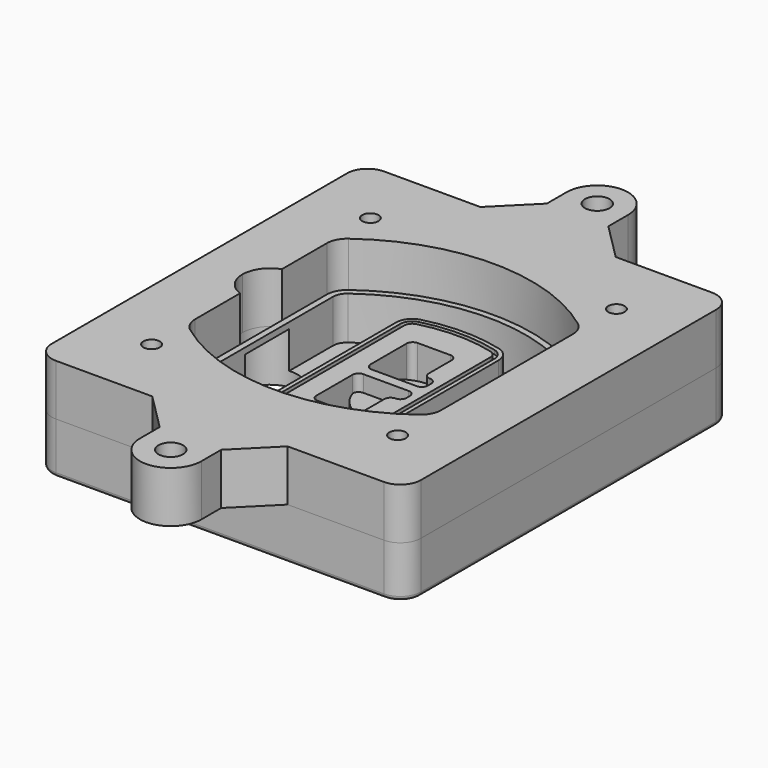
from build123d import *

# Parameters (mm, degrees)
F0_R      = 4
F1_DEPTH  = 25
F2_DEPTH  = 3
F3_DEPTH  = 18
F5_DEPTH  = 21
F6_DEPTH  = 2
F8_DEPTH  = 20
F9_DEPTH  = 16
F10_DEPTH = 25
F7_R      = 6
F7_R_2    = 4
F11_DEPTH = 6
F13_DEPTH = 9
F15_R     = 2
F16_R     = 4
F16_R_2   = 6
F17_DEPTH = 25


# Not quite as in the source:
# - a feature of the source that left no trace in its solid (it failed there, or was rolled back) is left out
# - a feature names something its author has since deleted; it is built from what else it names


with BuildPart() as f1:
    # F0 (on Top) → F1 (new body)
    with BuildSketch(Plane.XY):
        with BuildLine():
            ThreePointArc((-90, -90), (-87.0710678119, -97.0710678119), (-80, -100))
            Line((-80, -100), (80, -100))
            ThreePointArc((80, -100), (87.0710678119, -97.0710678119), (90, -90))
            Line((90, -90), (90, 90))
            ThreePointArc((90, 90), (87.0710678119, 97.0710678119), (80, 100))
            Line((80, 100), (-80, 100))
            ThreePointArc((-80, 100), (-87.0710678119, 97.0710678119), (-90, 90))
            Line((-90, 90), (-90, -90))
        make_face()
        with Locations((-60, -66.6666666667)):
            Circle(F0_R, mode=Mode.SUBTRACT)
        with Locations((60, -66.6666666667)):
            Circle(F0_R, mode=Mode.SUBTRACT)
        with Locations((-60, 66.6666666667)):
            Circle(F0_R, mode=Mode.SUBTRACT)
        with BuildLine():
            ThreePointArc((-64, 40.142841612), (-62.5058275186, 46.4360346072), (-58.3422459893, 51.3859253461))
            ThreePointArc((-58.3422459893, 51.3859253461), (0, 70.6666666667), (58.3422459893, 51.3859253461))
            ThreePointArc((58.3422459893, 51.3859253461), (62.5058275186, 46.4360346072), (64, 40.142841612))
            Line((64, 40.142841612), (64, -40.142841612))
            ThreePointArc((64, -40.142841612), (62.5058275186, -46.4360346072), (58.3422459893, -51.3859253461))
            ThreePointArc((58.3422459893, -51.3859253461), (0, -70.6666666667), (-58.3422459893, -51.3859253461))
            ThreePointArc((-58.3422459893, -51.3859253461), (-62.5058275186, -46.4360346072), (-64, -40.142841612))
            Line((-64, -40.142841612), (-64, 40.142841612))
        make_face(mode=Mode.SUBTRACT)
        with Locations((60, 66.6666666667)):
            Circle(F0_R, mode=Mode.SUBTRACT)
        with BuildLine():
            ThreePointArc((58.3422459893, 51.3859253461), (0, 70.6666666667), (-58.3422459893, 51.3859253461))
            ThreePointArc((-58.3422459893, 51.3859253461), (-62.5058275186, 46.4360346072), (-64, 40.142841612))
            Line((-64, 40.142841612), (-64, -40.142841612))
            ThreePointArc((-64, -40.142841612), (-62.5058275186, -46.4360346072), (-58.3422459893, -51.3859253461))
            ThreePointArc((-58.3422459893, -51.3859253461), (0, -70.6666666667), (58.3422459893, -51.3859253461))
            ThreePointArc((58.3422459893, -51.3859253461), (62.5058275186, -46.4360346072), (64, -40.142841612))
            Line((64, -40.142841612), (64, 40.142841612))
            ThreePointArc((64, 40.142841612), (62.5058275186, 46.4360346072), (58.3422459893, 51.3859253461))
        make_face()
        with BuildLine():
            Line((-60, -40.142841612), (-60, 40.142841612))
            ThreePointArc((-60, 40.142841612), (-58.9327339419, 44.6379794657), (-55.9587471352, 48.1736157078))
            ThreePointArc((-55.9587471352, 48.1736157078), (0, 66.6666666667), (55.9587471352, 48.1736157078))
            ThreePointArc((55.9587471352, 48.1736157078), (58.9327339419, 44.6379794657), (60, 40.142841612))
            Line((60, 40.142841612), (60, -40.142841612))
            ThreePointArc((60, -40.142841612), (58.9327339419, -44.6379794657), (55.9587471352, -48.1736157078))
            ThreePointArc((55.9587471352, -48.1736157078), (0, -66.6666666667), (-55.9587471352, -48.1736157078))
            ThreePointArc((-55.9587471352, -48.1736157078), (-58.9327339419, -44.6379794657), (-60, -40.142841612))
        make_face(mode=Mode.SUBTRACT)
        with BuildLine():
            ThreePointArc((-55.9587471352, 48.1736157078), (-58.9327339419, 44.6379794657), (-60, 40.142841612))
            Line((-60, 40.142841612), (-60, -40.142841612))
            ThreePointArc((-60, -40.142841612), (-58.9327339419, -44.6379794657), (-55.9587471352, -48.1736157078))
            ThreePointArc((-55.9587471352, -48.1736157078), (0, -66.6666666667), (55.9587471352, -48.1736157078))
            ThreePointArc((55.9587471352, -48.1736157078), (58.9327339419, -44.6379794657), (60, -40.142841612))
            Line((60, -40.142841612), (60, 40.142841612))
            ThreePointArc((60, 40.142841612), (58.9327339419, 44.6379794657), (55.9587471352, 48.1736157078))
            ThreePointArc((55.9587471352, 48.1736157078), (0, 66.6666666667), (-55.9587471352, 48.1736157078))
        make_face()
        with BuildLine():
            ThreePointArc((54.1711229947, 45.764383479), (56.2529137593, 43.2894381096), (57, 40.142841612))
            Line((57, 40.142841612), (57, -40.142841612))
            ThreePointArc((57, -40.142841612), (56.2529137593, -43.2894381096), (54.1711229947, -45.764383479))
            ThreePointArc((54.1711229947, -45.764383479), (0, -63.6666666667), (-54.1711229947, -45.764383479))
            ThreePointArc((-54.1711229947, -45.764383479), (-56.2529137593, -43.2894381096), (-57, -40.142841612))
            Line((-57, -40.142841612), (-57, 40.142841612))
            ThreePointArc((-57, 40.142841612), (-56.2529137593, 43.2894381096), (-54.1711229947, 45.764383479))
            ThreePointArc((-54.1711229947, 45.764383479), (0, 63.6666666667), (54.1711229947, 45.764383479))
        make_face(mode=Mode.SUBTRACT)
        with BuildLine():
            Line((57, -40.142841612), (57, 40.142841612))
            ThreePointArc((57, 40.142841612), (56.2529137593, 43.2894381096), (54.1711229947, 45.764383479))
            ThreePointArc((54.1711229947, 45.764383479), (0, 63.6666666667), (-54.1711229947, 45.764383479))
            ThreePointArc((-54.1711229947, 45.764383479), (-56.2529137593, 43.2894381096), (-57, 40.142841612))
            Line((-57, 40.142841612), (-57, -40.142841612))
            ThreePointArc((-57, -40.142841612), (-56.2529137593, -43.2894381096), (-54.1711229947, -45.764383479))
            ThreePointArc((-54.1711229947, -45.764383479), (0, -63.6666666667), (54.1711229947, -45.764383479))
            ThreePointArc((54.1711229947, -45.764383479), (56.2529137593, -43.2894381096), (57, -40.142841612))
        make_face()
    extrude(amount=-F1_DEPTH)

    # F0 (on Top) → F2 (join)
    with BuildSketch(Plane.XY):
        with BuildLine():
            ThreePointArc((-55.9587471352, 48.1736157078), (-58.9327339419, 44.6379794657), (-60, 40.142841612))
            Line((-60, 40.142841612), (-60, -40.142841612))
            ThreePointArc((-60, -40.142841612), (-58.9327339419, -44.6379794657), (-55.9587471352, -48.1736157078))
            ThreePointArc((-55.9587471352, -48.1736157078), (0, -66.6666666667), (55.9587471352, -48.1736157078))
            ThreePointArc((55.9587471352, -48.1736157078), (58.9327339419, -44.6379794657), (60, -40.142841612))
            Line((60, -40.142841612), (60, 40.142841612))
            ThreePointArc((60, 40.142841612), (58.9327339419, 44.6379794657), (55.9587471352, 48.1736157078))
            ThreePointArc((55.9587471352, 48.1736157078), (0, 66.6666666667), (-55.9587471352, 48.1736157078))
        make_face()
        with BuildLine():
            ThreePointArc((54.1711229947, 45.764383479), (56.2529137593, 43.2894381096), (57, 40.142841612))
            Line((57, 40.142841612), (57, -40.142841612))
            ThreePointArc((57, -40.142841612), (56.2529137593, -43.2894381096), (54.1711229947, -45.764383479))
            ThreePointArc((54.1711229947, -45.764383479), (0, -63.6666666667), (-54.1711229947, -45.764383479))
            ThreePointArc((-54.1711229947, -45.764383479), (-56.2529137593, -43.2894381096), (-57, -40.142841612))
            Line((-57, -40.142841612), (-57, 40.142841612))
            ThreePointArc((-57, 40.142841612), (-56.2529137593, 43.2894381096), (-54.1711229947, 45.764383479))
            ThreePointArc((-54.1711229947, 45.764383479), (0, 63.6666666667), (54.1711229947, 45.764383479))
        make_face(mode=Mode.SUBTRACT)
    extrude(amount=F2_DEPTH)

    # F0 (on Top) → F3 (cut)
    with BuildSketch(Plane.XY):
        with BuildLine():
            Line((57, -40.142841612), (57, 40.142841612))
            ThreePointArc((57, 40.142841612), (56.2529137593, 43.2894381096), (54.1711229947, 45.764383479))
            ThreePointArc((54.1711229947, 45.764383479), (0, 63.6666666667), (-54.1711229947, 45.764383479))
            ThreePointArc((-54.1711229947, 45.764383479), (-56.2529137593, 43.2894381096), (-57, 40.142841612))
            Line((-57, 40.142841612), (-57, -40.142841612))
            ThreePointArc((-57, -40.142841612), (-56.2529137593, -43.2894381096), (-54.1711229947, -45.764383479))
            ThreePointArc((-54.1711229947, -45.764383479), (0, -63.6666666667), (54.1711229947, -45.764383479))
            ThreePointArc((54.1711229947, -45.764383479), (56.2529137593, -43.2894381096), (57, -40.142841612))
        make_face()
    extrude(amount=-F3_DEPTH, mode=Mode.SUBTRACT)

    # F4 (on face) → F5 (join, through all)
    with BuildSketch(Plane.XY.offset(3)):
        with BuildLine():
            ThreePointArc((-25, -38.5044362778), (-23.3253910568, -43.402336642), (-19.0026430055, -46.2497200681))
            ThreePointArc((-19.0026430055, -46.2497200681), (0, -48.6666666667), (19.0026430055, -46.2497200681))
            ThreePointArc((19.0026430055, -46.2497200681), (23.3253910568, -43.402336642), (25, -38.5044362778))
            Line((25, -38.5044362778), (25, 38.5044362778))
            ThreePointArc((25, 38.5044362778), (23.3253910568, 43.402336642), (19.0026430055, 46.2497200681))
            ThreePointArc((19.0026430055, 46.2497200681), (0, 48.6666666667), (-19.0026430055, 46.2497200681))
            ThreePointArc((-19.0026430055, 46.2497200681), (-23.3253910568, 43.402336642), (-25, 38.5044362778))
            Line((-25, 38.5044362778), (-25, -38.5044362778))
        make_face()
        with BuildLine():
            ThreePointArc((18.5019822541, 44.3133991205), (21.7440432926, 42.177861551), (23, 38.5044362778))
            Line((23, 38.5044362778), (23, -38.5044362778))
            ThreePointArc((23, -38.5044362778), (21.7440432926, -42.177861551), (18.5019822541, -44.3133991205))
            ThreePointArc((18.5019822541, -44.3133991205), (0, -46.6666666667), (-18.5019822541, -44.3133991205))
            ThreePointArc((-18.5019822541, -44.3133991205), (-21.7440432926, -42.177861551), (-23, -38.5044362778))
            Line((-23, -38.5044362778), (-23, 38.5044362778))
            ThreePointArc((-23, 38.5044362778), (-21.7440432926, 42.177861551), (-18.5019822541, 44.3133991205))
            ThreePointArc((-18.5019822541, 44.3133991205), (0, 46.6666666667), (18.5019822541, 44.3133991205))
        make_face(mode=Mode.SUBTRACT)
        with BuildLine():
            Line((23, -38.5044362778), (23, 38.5044362778))
            ThreePointArc((23, 38.5044362778), (21.7440432926, 42.177861551), (18.5019822541, 44.3133991205))
            ThreePointArc((18.5019822541, 44.3133991205), (0, 46.6666666667), (-18.5019822541, 44.3133991205))
            ThreePointArc((-18.5019822541, 44.3133991205), (-21.7440432926, 42.177861551), (-23, 38.5044362778))
            Line((-23, 38.5044362778), (-23, -38.5044362778))
            ThreePointArc((-23, -38.5044362778), (-21.7440432926, -42.177861551), (-18.5019822541, -44.3133991205))
            ThreePointArc((-18.5019822541, -44.3133991205), (0, -46.6666666667), (18.5019822541, -44.3133991205))
            ThreePointArc((18.5019822541, -44.3133991205), (21.7440432926, -42.177861551), (23, -38.5044362778))
        make_face()
        with BuildLine():
            ThreePointArc((18.0013215027, 42.3770781729), (20.1626955284, 40.9533864599), (21, 38.5044362778))
            Line((21, 38.5044362778), (21, -38.5044362778))
            ThreePointArc((21, -38.5044362778), (20.1626955284, -40.9533864599), (18.0013215027, -42.3770781729))
            ThreePointArc((18.0013215027, -42.3770781729), (0, -44.6666666667), (-18.0013215027, -42.3770781729))
            ThreePointArc((-18.0013215027, -42.3770781729), (-20.1626955284, -40.9533864599), (-21, -38.5044362778))
            Line((-21, -38.5044362778), (-21, 38.5044362778))
            ThreePointArc((-21, 38.5044362778), (-20.1626955284, 40.9533864599), (-18.0013215027, 42.3770781729))
            ThreePointArc((-18.0013215027, 42.3770781729), (0, 44.6666666667), (18.0013215027, 42.3770781729))
        make_face(mode=Mode.SUBTRACT)
        with BuildLine():
            Line((21, -38.5044362778), (21, 38.5044362778))
            ThreePointArc((21, 38.5044362778), (20.1626955284, 40.9533864599), (18.0013215027, 42.3770781729))
            ThreePointArc((18.0013215027, 42.3770781729), (0, 44.6666666667), (-18.0013215027, 42.3770781729))
            ThreePointArc((-18.0013215027, 42.3770781729), (-20.1626955284, 40.9533864599), (-21, 38.5044362778))
            Line((-21, 38.5044362778), (-21, -38.5044362778))
            ThreePointArc((-21, -38.5044362778), (-20.1626955284, -40.9533864599), (-18.0013215027, -42.3770781729))
            ThreePointArc((-18.0013215027, -42.3770781729), (0, -44.6666666667), (18.0013215027, -42.3770781729))
            ThreePointArc((18.0013215027, -42.3770781729), (20.1626955284, -40.9533864599), (21, -38.5044362778))
        make_face()
        with BuildLine():
            Line((-8, -2.5), (14, -2.5))
            ThreePointArc((14, -2.5), (16.1213203436, -3.3786796564), (17, -5.5))
            Line((17, -5.5), (17, -7.5))
            ThreePointArc((17, -7.5), (16.1213203436, -9.6213203436), (14, -10.5))
            ThreePointArc((14, -10.5), (11.8786796564, -11.3786796564), (11, -13.5))
            Line((11, -13.5), (11, -27.5))
            ThreePointArc((11, -27.5), (10.1213203436, -29.6213203436), (8, -30.5))
            Line((8, -30.5), (-8, -30.5))
            ThreePointArc((-8, -30.5), (-10.1213203436, -29.6213203436), (-11, -27.5))
            Line((-11, -27.5), (-11, -5.5))
            ThreePointArc((-11, -5.5), (-10.1213203436, -3.3786796564), (-8, -2.5))
        make_face(mode=Mode.SUBTRACT)
        with BuildLine():
            ThreePointArc((-8, 2.5), (-10.1213203436, 3.3786796564), (-11, 5.5))
            Line((-11, 5.5), (-11, 27.5))
            ThreePointArc((-11, 27.5), (-10.1213203436, 29.6213203436), (-8, 30.5))
            Line((-8, 30.5), (8, 30.5))
            ThreePointArc((8, 30.5), (10.1213203436, 29.6213203436), (11, 27.5))
            Line((11, 27.5), (11, 13.5))
            ThreePointArc((11, 13.5), (11.8786796564, 11.3786796564), (14, 10.5))
            ThreePointArc((14, 10.5), (16.1213203436, 9.6213203436), (17, 7.5))
            Line((17, 7.5), (17, 5.5))
            ThreePointArc((17, 5.5), (16.1213203436, 3.3786796564), (14, 2.5))
            Line((14, 2.5), (-8, 2.5))
        make_face(mode=Mode.SUBTRACT)
    extrude(amount=-F5_DEPTH)

    # F4 (on face) → F6 (cut)
    with BuildSketch(Plane.XY.offset(3)):
        with BuildLine():
            Line((23, -38.5044362778), (23, 38.5044362778))
            ThreePointArc((23, 38.5044362778), (21.7440432926, 42.177861551), (18.5019822541, 44.3133991205))
            ThreePointArc((18.5019822541, 44.3133991205), (0, 46.6666666667), (-18.5019822541, 44.3133991205))
            ThreePointArc((-18.5019822541, 44.3133991205), (-21.7440432926, 42.177861551), (-23, 38.5044362778))
            Line((-23, 38.5044362778), (-23, -38.5044362778))
            ThreePointArc((-23, -38.5044362778), (-21.7440432926, -42.177861551), (-18.5019822541, -44.3133991205))
            ThreePointArc((-18.5019822541, -44.3133991205), (0, -46.6666666667), (18.5019822541, -44.3133991205))
            ThreePointArc((18.5019822541, -44.3133991205), (21.7440432926, -42.177861551), (23, -38.5044362778))
        make_face()
        with BuildLine():
            ThreePointArc((18.0013215027, 42.3770781729), (20.1626955284, 40.9533864599), (21, 38.5044362778))
            Line((21, 38.5044362778), (21, -38.5044362778))
            ThreePointArc((21, -38.5044362778), (20.1626955284, -40.9533864599), (18.0013215027, -42.3770781729))
            ThreePointArc((18.0013215027, -42.3770781729), (0, -44.6666666667), (-18.0013215027, -42.3770781729))
            ThreePointArc((-18.0013215027, -42.3770781729), (-20.1626955284, -40.9533864599), (-21, -38.5044362778))
            Line((-21, -38.5044362778), (-21, 38.5044362778))
            ThreePointArc((-21, 38.5044362778), (-20.1626955284, 40.9533864599), (-18.0013215027, 42.3770781729))
            ThreePointArc((-18.0013215027, 42.3770781729), (0, 44.6666666667), (18.0013215027, 42.3770781729))
        make_face(mode=Mode.SUBTRACT)
    extrude(amount=-F6_DEPTH, mode=Mode.SUBTRACT)

    # F7 (on face) → F8 (join)
    with BuildSketch(Plane(origin=(0, 0, -25), x_dir=(1, 0, 0), z_dir=(0, 0, -1))):
        with BuildLine():
            ThreePointArc((-6.71157564, 0), (6.7567035675, 13.4682792075), (20.224982775, 0))
            Line((20.224982775, 0), (25.224982775, 0))
            ThreePointArc((25.224982775, 0), (6.7567035675, 18.4682792075), (-11.71157564, 0))
            Line((-11.71157564, 0), (-6.71157564, 0))
        make_face()
        with BuildLine():
            Line((-6.71157564, 0), (20.224982775, 0))
            ThreePointArc((20.224982775, 0), (6.7567035675, 13.4682792075), (-6.71157564, 0))
        make_face()
        with BuildLine():
            ThreePointArc((-6.71157564, 0), (6.7567035675, -13.4682792075), (20.224982775, 0))
            Line((20.224982775, 0), (-6.71157564, 0))
        make_face()
        with BuildLine():
            Line((25.224982775, 0), (20.224982775, 0))
            ThreePointArc((20.224982775, 0), (6.7567035675, -13.4682792075), (-6.71157564, 0))
            Line((-6.71157564, 0), (-11.71157564, 0))
            ThreePointArc((-11.71157564, 0), (6.7567035675, -18.4682792075), (25.224982775, 0))
        make_face()
    extrude(amount=-F8_DEPTH)

    # F7 (on face) → F9 (cut)
    with BuildSketch(Plane(origin=(0, 0, -25), x_dir=(1, 0, 0), z_dir=(0, 0, -1))):
        with BuildLine():
            Line((-6.71157564, 0), (20.224982775, 0))
            ThreePointArc((20.224982775, 0), (6.7567035675, 13.4682792075), (-6.71157564, 0))
        make_face()
        with BuildLine():
            ThreePointArc((-6.71157564, 0), (6.7567035675, -13.4682792075), (20.224982775, 0))
            Line((20.224982775, 0), (-6.71157564, 0))
        make_face()
    extrude(amount=-F9_DEPTH, mode=Mode.SUBTRACT)

    # F7 (on face) → F10 (cut)
    with BuildSketch(Plane(origin=(0, 0, -25), x_dir=(1, 0, 0), z_dir=(0, 0, -1))):
        with BuildLine():
            Line((-69.0318229325, 0), (-42.0952645175, 0))
            ThreePointArc((-42.0952645175, 0), (-55.563543725, 13.4682792075), (-69.0318229325, 0))
        make_face()
        with BuildLine():
            ThreePointArc((-69.0318229325, 0), (-55.563543725, -13.4682792075), (-42.0952645175, 0))
            Line((-42.0952645175, 0), (-69.0318229325, 0))
        make_face()
    extrude(amount=-F10_DEPTH, mode=Mode.SUBTRACT)

    # F7 (on face) → F11 (cut)
    with BuildSketch(Plane(origin=(0, 0, -25), x_dir=(1, 0, 0), z_dir=(0, 0, -1))):
        with Locations((60, -66.6666666667)):
            Circle(F7_R)
        with Locations((60, -66.6666666667)):
            Circle(F7_R_2, mode=Mode.SUBTRACT)
        with Locations((-60, -66.6666666667)):
            Circle(F7_R)
        with Locations((-60, -66.6666666667)):
            Circle(F7_R_2, mode=Mode.SUBTRACT)
        with Locations((-60, 66.6666666667)):
            Circle(F7_R)
        with Locations((-60, 66.6666666667)):
            Circle(F7_R_2, mode=Mode.SUBTRACT)
        with Locations((60, 66.6666666667)):
            Circle(F7_R)
        with Locations((60, 66.6666666667)):
            Circle(F7_R_2, mode=Mode.SUBTRACT)
    extrude(amount=-F11_DEPTH, mode=Mode.SUBTRACT)

    # F12 (on face) → F13 (cut, through all)
    with BuildSketch(Plane(origin=(0, 0, -9), x_dir=(1, 0, 0), z_dir=(0, 0, -1))):
        with BuildLine():
            ThreePointArc((20.224982775, 0), (20.1663399806, 1.2554664788), (19.9909222755, 2.5))
            Line((19.9909222755, 2.5), (14, 2.5))
            ThreePointArc((14, 2.5), (16.1213203436, 3.3786796564), (17, 5.5))
            Line((17, 5.5), (17, 7.5))
            ThreePointArc((17, 7.5), (16.1213203436, 9.6213203436), (14, 10.5))
            ThreePointArc((14, 10.5), (12.1627255951, 11.1284134507), (11.0951631559, 12.750384826))
            ThreePointArc((11.0951631559, 12.750384826), (11.0476113807, 12.7664660322), (11, 12.7823698976))
            Line((11, 12.7823698976), (11, -12.7823698976))
            ThreePointArc((11, -12.7823698976), (11.0476113807, -12.7664660322), (11.0951631559, -12.750384826))
            ThreePointArc((11.0951631559, -12.750384826), (12.1627255951, -11.1284134507), (14, -10.5))
            ThreePointArc((14, -10.5), (16.1213203436, -9.6213203436), (17, -7.5))
            Line((17, -7.5), (17, -5.5))
            ThreePointArc((17, -5.5), (16.1213203436, -3.3786796564), (14, -2.5))
            Line((14, -2.5), (19.9909222755, -2.5))
            ThreePointArc((19.9909222755, -2.5), (20.1663399806, -1.2554664788), (20.224982775, 0))
        make_face()
    extrude(amount=F13_DEPTH, mode=Mode.SUBTRACT)

    # F15
    f15_edges = [f1.edges().sort_by_distance(p)[0] for p in [
        (0, -100, -25),
        (-87.071068, -97.071068, -25),
        (-90, 0, -25),
        (-87.071068, 97.071068, -25),
        (87.071068, -97.071068, -25),
        (0, 100, -25),
        (90, 0, -25),
        (87.071068, 97.071068, -25),
    ]]
    fillet(f15_edges, radius=F15_R)


with BuildPart() as f17:
    # F16 (on face) → F17 (new body)
    with BuildSketch(Plane.XY):
        with BuildLine():
            Line((33, 100), (-33, 100))
            Line((-33, 100), (-80, 100))
            ThreePointArc((-80, 100), (-87.0710678119, 97.0710678119), (-90, 90))
            Line((-90, 90), (-90, -90))
            ThreePointArc((-90, -90), (-87.0710678119, -97.0710678119), (-80, -100))
            Line((-80, -100), (-33, -100))
            Line((-33, -100), (33, -100))
            Line((33, -100), (80, -100))
            ThreePointArc((80, -100), (87.0710678119, -97.0710678119), (90, -90))
            Line((90, -90), (90, 90))
            ThreePointArc((90, 90), (87.0710678119, 97.0710678119), (80, 100))
            Line((80, 100), (33, 100))
        make_face()
        with Locations((-60, -66.6666666667)):
            Circle(F16_R, mode=Mode.SUBTRACT)
        with Locations((60, -66.6666666667)):
            Circle(F16_R, mode=Mode.SUBTRACT)
        with Locations((-60, 66.6666666667)):
            Circle(F16_R, mode=Mode.SUBTRACT)
        with BuildLine():
            ThreePointArc((-60, 40.142841612), (-58.9327339419, 44.6379794657), (-55.9587471352, 48.1736157078))
            ThreePointArc((-55.9587471352, 48.1736157078), (0, 66.6666666667), (55.9587471352, 48.1736157078))
            ThreePointArc((55.9587471352, 48.1736157078), (58.9327339419, 44.6379794657), (60, 40.142841612))
            Line((60, 40.142841612), (60, -40.142841612))
            ThreePointArc((60, -40.142841612), (58.9327339419, -44.6379794657), (55.9587471352, -48.1736157078))
            ThreePointArc((55.9587471352, -48.1736157078), (0, -66.6666666667), (-55.9587471352, -48.1736157078))
            ThreePointArc((-55.9587471352, -48.1736157078), (-58.9327339419, -44.6379794657), (-60, -40.142841612))
            Line((-60, -40.142841612), (-60, -12.7166190685))
            ThreePointArc((-60, -12.7166190685), (-66.5441169481, -7.798817635), (-69.0318229325, 0))
            ThreePointArc((-69.0318229325, 0), (-66.5441169481, 7.798817635), (-60, 12.7166190685))
            Line((-60, 12.7166190685), (-60, 40.142841612))
        make_face(mode=Mode.SUBTRACT)
        with Locations((60, 66.6666666667)):
            Circle(F16_R, mode=Mode.SUBTRACT)
        with BuildLine():
            Line((-15, 118), (-33, 100))
            Line((-33, 100), (33, 100))
            Line((33, 100), (15, 118))
            Line((15, 118), (15, 130))
            ThreePointArc((15, 130), (0, 145), (-15, 130))
            Line((-15, 130), (-15, 118))
        make_face()
        with Locations((0, 130)):
            Circle(F16_R_2, mode=Mode.SUBTRACT)
        with BuildLine():
            Line((33, -100), (-33, -100))
            Line((-33, -100), (-15, -118))
            Line((-15, -118), (-15, -130))
            ThreePointArc((-15, -130), (0, -145), (15, -130))
            Line((15, -130), (15, -118))
            Line((15, -118), (33, -100))
        make_face()
        with Locations((0, -130)):
            Circle(F16_R_2, mode=Mode.SUBTRACT)
    extrude(amount=F17_DEPTH)


solid = Compound([f1.part, f17.part])
